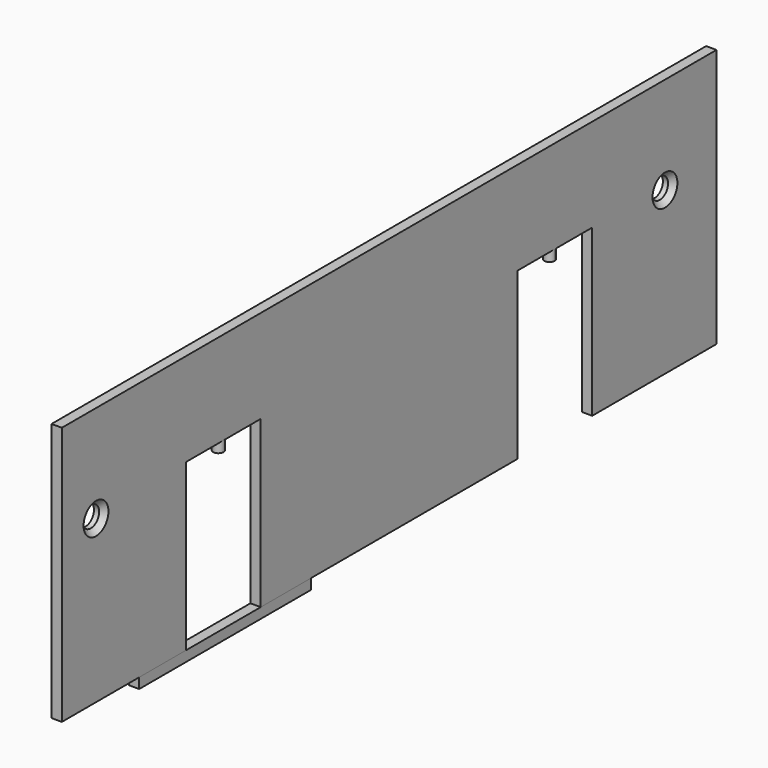
from build123d import *

# Parameters (mm, degrees)
F1_DEPTH       = 1
F3_D           = 2
F3_CSINK_D     = 3
F3_CSINK_ANGLE = 90
F5_DEPTH       = 1
F7_DEPTH       = 1
F8_W           = 1
F8_H           = 20.7052147016
F9_DEPTH       = 1


with BuildPart() as f1:
    # F0 (on Right) → F1 (new body)
    with BuildSketch(Plane.YZ):
        Polygon((40.680675586, 25), (-38.319324414, 25), (-38.319324414, 0), (-23.319324414, 0), (-23.319324414, 16), (-14.319324414, 16), (-14.319324414, 0), (16.680675586, 0), (16.680675586, 16), (25.680675586, 16), (25.680675586, 0), (40.680675586, 0), align=None)
    extrude(amount=F1_DEPTH)

    # F3 (through all)
    with Locations(Plane.YZ.offset(1)):
        with Locations((-34.1976433992, 15.6130259857), (34.4599224627, 15.6130259857)):
            CounterSinkHole(F3_D / 2, F3_CSINK_D / 2, counter_sink_angle=F3_CSINK_ANGLE)

    # F4 (on face) → F5 (join)
    with BuildSketch(Plane(origin=(0, 0, 16), x_dir=(1, 0, 0), z_dir=(0, 0, -1))):
        with BuildLine():
            ThreePointArc((-8.68652e-05, 18.8100038602), (0.5, 18.309916995), (1.0000868652, 18.8100038602))
            ThreePointArc((1.0000868652, 18.8100038602), (0.5, 19.3100907254), (-8.68652e-05, 18.8100038602))
        make_face()
    extrude(amount=F5_DEPTH)

    # F6 (on face) → F7 (join)
    with BuildSketch(Plane(origin=(0, 0, 16), x_dir=(1, 0, 0), z_dir=(0, 0, -1))):
        with BuildLine():
            Line((1, -21.180675586), (1, -21.1288443983))
            ThreePointArc((1, -21.1288443983), (0.5, -20.6540888246), (0, -21.1288443983))
            Line((0, -21.1288443983), (0, -21.180675586))
            ThreePointArc((0, -21.180675586), (0.5, -21.6554311597), (1, -21.180675586))
        make_face()
    extrude(amount=F7_DEPTH)


with BuildPart() as f9:
    # F8 (on face) → F9 (new body)
    with BuildSketch(Plane(origin=(0, 0, 0), x_dir=(1, 0, 0), z_dir=(0, 0, -1))):
        with Locations((0.5, 18.6329078861)):
            Rectangle(F8_W, F8_H)
    extrude(amount=F9_DEPTH)


solid = Compound([f1.part, f9.part])
